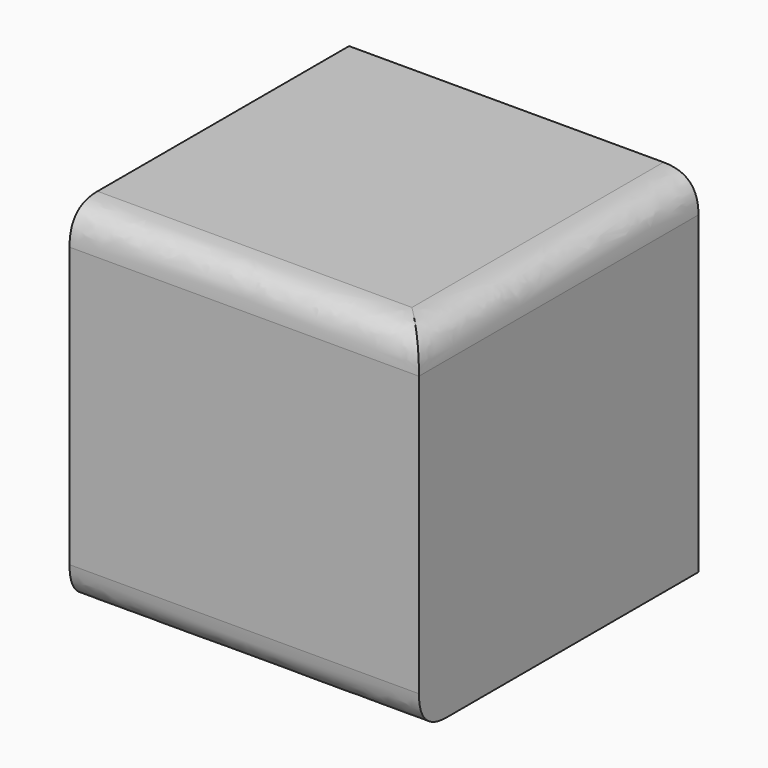
from build123d import *

# Parameters (mm, degrees)
F0_W        = 50.8
F0_H        = 50.8
F1_DEPTH    = 50.8
F2_T1_DEPTH = 76.2
F2_T3_DEPTH = 76.2
F3_T1_DEPTH = 76.2


# Not quite as in the source:
# - a fillet or chamfer that OpenCascade refuses, or shapes differently, is made with other operations: its cross-section is extruded or revolved along the edge and cut away or added


with BuildPart() as f1:
    # F0 (on Front) → F1 (new body)
    with BuildSketch(Plane.XZ):
        with Locations((25.4, 25.4)):
            Rectangle(F0_W, F0_H)
    extrude(amount=F1_DEPTH)

    # F2: fillet of radius 5.08 on 2 edges, made by hand

    # F2_s2 → F2_t1 (cut)
    with BuildSketch(Plane.XZ.offset(-12.7)):
        with BuildLine():
            add(Edge.make_bspline(
                [(50.8, 45.72), (50.8, 50.8), (45.72, 50.8)],
                knots=[0, 0, 0, 1, 1, 1], degree=2, weights=[1, 1, 1]))
            Line((45.72, 50.8), (50.8, 50.8))
            Line((50.8, 50.8), (50.8, 45.72))
        make_face()
    extrude(amount=F2_T1_DEPTH, mode=Mode.SUBTRACT)

    # F2_s4 → F2_t3 (cut)
    with BuildSketch(Plane.YZ.offset(-12.7)):
        with BuildLine():
            add(Edge.make_bspline(
                [(-45.72, 50.8), (-50.8, 50.8), (-50.8, 45.72)],
                knots=[0, 0, 0, 1, 1, 1], degree=2, weights=[1, 1, 1]))
            Line((-50.8, 45.72), (-50.8, 50.8))
            Line((-50.8, 50.8), (-45.72, 50.8))
        make_face()
    extrude(amount=F2_T3_DEPTH, mode=Mode.SUBTRACT)

    # F3: fillet of radius 5.08 on 1 edges, made by hand

    # F3_s2 → F3_t1 (cut)
    with BuildSketch(Plane.YZ.offset(-12.7)):
        with BuildLine():
            add(Edge.make_bspline(
                [(-45.72, 0), (-50.8, 0), (-50.8, 5.08)],
                knots=[0, 0, 0, 1, 1, 1], degree=2, weights=[1, 1, 1]))
            Line((-50.8, 5.08), (-50.8, 0))
            Line((-50.8, 0), (-45.72, 0))
        make_face()
    extrude(amount=F3_T1_DEPTH, mode=Mode.SUBTRACT)


solid = f1.part
